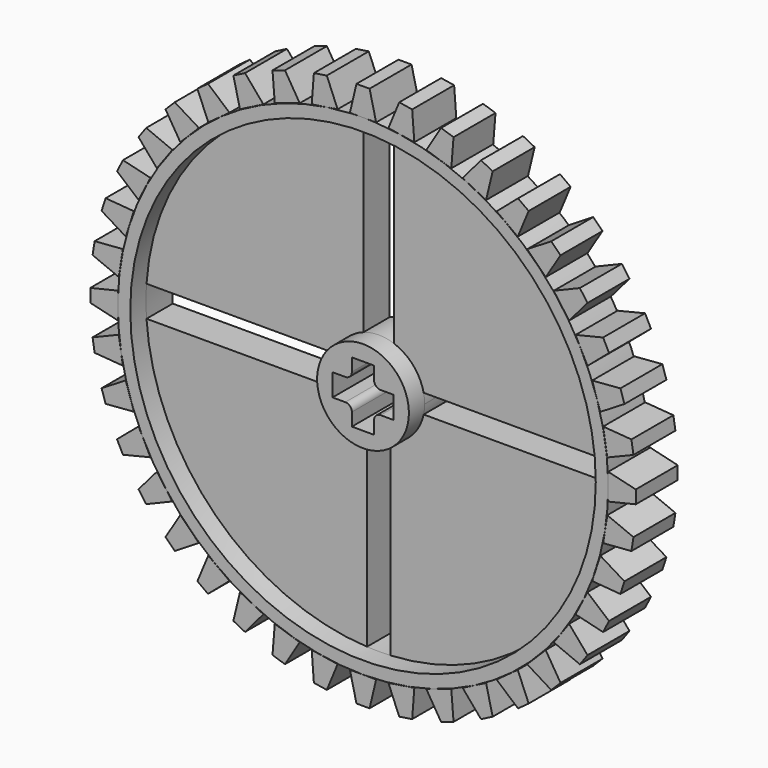
from build123d import *

# Parameters (mm, degrees)
F1_DEPTH        = 4
F2_DEPTH        = 4
F2_COPIES_COUNT = 40
F3_W            = 1.475
F3_H            = 1.693
F3_W_2          = 1.693
F3_H_2          = 1.4767124441
F3_W_3          = 1.482
F3_H_3          = 1.4802875559
F4_DEPTH        = 25
F5_R            = 17.75
F5_R_2          = 3.5
F6_DEPTH        = 0.75
F7_R            = 17.75
F7_R_2          = 3.5
F8_DEPTH        = 0.75
F9_R            = 0.5
F11_DEPTH       = 25


# Not quite as in the source:
# - after a boolean that leaves OpenCascade's solid faulty, fix() repairs it
# - a pattern or mirror of a feature is missing from the dataset's text; its kind, count and spacing are read off the source's solid


with BuildPart() as f1:
    # F0 (on Front) → F1 (new body)
    with BuildSketch(Plane.XZ):
        with BuildLine():
            ThreePointArc((-1.0015409707, 18.6731603025), (-12.8639259919, -13.5723766554), (18.7, 0))
            ThreePointArc((18.7, 0), (13.571937199, 12.8643896344), (1.0002651695, 18.6732286868))
            ThreePointArc((1.0002651695, 18.6732286868), (0.500311681, 18.6933059736), (0, 18.7))
            ThreePointArc((0, 18.7), (-0.5009502683, 18.6932888714), (-1.0015409707, 18.6731603025))
        make_face()
    extrude(amount=F1_DEPTH)

    # F3 (on face) → F4 (cut)
    with BuildSketch(Plane.XZ.offset(4)):
        with Locations((-1.5875, 0.0017875559)):
            Rectangle(F3_W, F3_H)
        with Locations((-0.0035, 1.5866437779)):
            Rectangle(F3_W_2, F3_H_2)
        with Locations((-0.0035, 0.0017875559)):
            Rectangle(F3_W_2, F3_H)
        with Locations((1.584, 0.0017875559)):
            Rectangle(F3_W_3, F3_H)
        with Locations((-0.0035, -1.5848562221)):
            Rectangle(F3_W_2, F3_H_3)
    extrude(amount=-F4_DEPTH, mode=Mode.SUBTRACT)

    # F5 (on face) → F6 (cut)
    with BuildSketch(Plane.XZ.offset(4)):
        Circle(F5_R)
        Circle(F5_R_2, mode=Mode.SUBTRACT)
    extrude(amount=-F6_DEPTH, mode=Mode.SUBTRACT)

    # F7 (on face) → F8 (cut)
    with BuildSketch(Plane.XZ.offset(3.25)):
        Circle(F7_R)
        Circle(F7_R_2, mode=Mode.SUBTRACT)
    extrude(amount=-F8_DEPTH, mode=Mode.SUBTRACT)

    # F9
    f9_edges = [f1.edges().sort_by_distance(p)[0] for p in [
        (-0.85, -2, 0.848288),
        (0.843, -2, 0.848288),
        (-0.85, -2, -0.844712),
        (0.843, -2, -0.844712),
    ]]
    fillet(f9_edges, radius=F9_R)

    # F10 (on face) → F11 (cut)
    with BuildSketch(Plane.XZ.offset(2.5)):
        with BuildLine():
            ThreePointArc((-3.2968505322, -1.1750644953), (-3.5, 0), (-3.2968505322, 1.1750644953))
            Line((-3.2968505322, 1.1750644953), (-17.7110621768, 1.1750644953))
            ThreePointArc((-17.7110621768, 1.1750644953), (-17.75, 0), (-17.7110621768, -1.1750644953))
            Line((-17.7110621768, -1.1750644953), (-3.2968505322, -1.1750644953))
        make_face()
        with BuildLine():
            Line((0.8961235281, -17.7273647963), (0.8961235281, -3.3833360197))
            ThreePointArc((0.8961235281, -3.3833360197), (0, -3.5), (-0.8961235281, -3.3833360197))
            Line((-0.8961235281, -3.3833360197), (-0.8961235281, -17.7273647963))
            ThreePointArc((-0.8961235281, -17.7273647963), (0, -17.75), (0.8961235281, -17.7273647963))
        make_face()
        with BuildLine():
            Line((17.7349775585, 0.7301171139), (3.423, 0.7301171139))
            ThreePointArc((3.423, 0.7301171139), (3.4806967693, 0.3670830969), (3.5, 0))
            ThreePointArc((3.5, 0), (3.4806967693, -0.3670830969), (3.423, -0.7301171139))
            Line((3.423, -0.7301171139), (17.7349775585, -0.7301171139))
            ThreePointArc((17.7349775585, -0.7301171139), (17.7462439922, -0.3651358219), (17.75, 0))
            ThreePointArc((17.75, 0), (17.7462439922, 0.3651358219), (17.7349775585, 0.7301171139))
        make_face()
        with BuildLine():
            ThreePointArc((-1.163931855, 3.3007972729), (0, 3.5), (1.163931855, 3.3007972729))
            Line((1.163931855, 3.3007972729), (1.163931855, 17.7117972729))
            ThreePointArc((1.163931855, 17.7117972729), (0, 17.75), (-1.163931855, 17.7117972729))
            Line((-1.163931855, 17.7117972729), (-1.163931855, 3.3007972729))
        make_face()
    extrude(amount=-F11_DEPTH, mode=Mode.SUBTRACT)

    add(f1.part.fix(), mode=Mode.REPLACE)


with BuildPart() as f2:
    # F0 (on Front) → F2 (new body)
    with BuildSketch(Plane.XZ):
        Polygon((-1, 18.7), (0, 18.7), (0, 20.8), (-0.5, 20.8), align=None)
        Polygon((0, 20.8), (0, 18.7), (1, 18.7), (0.5, 20.8), align=None)
    extrude(amount=F2_DEPTH)


with BuildPart() as f2_copies_1:
    # F2_copies: instance of F2
    add(f2.part.rotate(Axis((0, 0, 0), (0, 1, 0)), 1 * 360 / F2_COPIES_COUNT))


with BuildPart() as f2_copies_2:
    # F2_copies: instance of F2
    add(f2.part.rotate(Axis((0, 0, 0), (0, 1, 0)), 2 * 360 / F2_COPIES_COUNT))


with BuildPart() as f2_copies_3:
    # F2_copies: instance of F2
    add(f2.part.rotate(Axis((0, 0, 0), (0, 1, 0)), 3 * 360 / F2_COPIES_COUNT))


with BuildPart() as f2_copies_4:
    # F2_copies: instance of F2
    add(f2.part.rotate(Axis((0, 0, 0), (0, 1, 0)), 4 * 360 / F2_COPIES_COUNT))


with BuildPart() as f2_copies_5:
    # F2_copies: instance of F2
    add(f2.part.rotate(Axis((0, 0, 0), (0, 1, 0)), 5 * 360 / F2_COPIES_COUNT))


with BuildPart() as f2_copies_6:
    # F2_copies: instance of F2
    add(f2.part.rotate(Axis((0, 0, 0), (0, 1, 0)), 6 * 360 / F2_COPIES_COUNT))


with BuildPart() as f2_copies_7:
    # F2_copies: instance of F2
    add(f2.part.rotate(Axis((0, 0, 0), (0, 1, 0)), 7 * 360 / F2_COPIES_COUNT))


with BuildPart() as f2_copies_8:
    # F2_copies: instance of F2
    add(f2.part.rotate(Axis((0, 0, 0), (0, 1, 0)), 8 * 360 / F2_COPIES_COUNT))


with BuildPart() as f2_copies_9:
    # F2_copies: instance of F2
    add(f2.part.rotate(Axis((0, 0, 0), (0, 1, 0)), 9 * 360 / F2_COPIES_COUNT))


with BuildPart() as f2_copies_10:
    # F2_copies: instance of F2
    add(f2.part.rotate(Axis((0, 0, 0), (0, 1, 0)), 10 * 360 / F2_COPIES_COUNT))


with BuildPart() as f2_copies_11:
    # F2_copies: instance of F2
    add(f2.part.rotate(Axis((0, 0, 0), (0, 1, 0)), 11 * 360 / F2_COPIES_COUNT))


with BuildPart() as f2_copies_12:
    # F2_copies: instance of F2
    add(f2.part.rotate(Axis((0, 0, 0), (0, 1, 0)), 12 * 360 / F2_COPIES_COUNT))


with BuildPart() as f2_copies_13:
    # F2_copies: instance of F2
    add(f2.part.rotate(Axis((0, 0, 0), (0, 1, 0)), 13 * 360 / F2_COPIES_COUNT))


with BuildPart() as f2_copies_14:
    # F2_copies: instance of F2
    add(f2.part.rotate(Axis((0, 0, 0), (0, 1, 0)), 14 * 360 / F2_COPIES_COUNT))


with BuildPart() as f2_copies_15:
    # F2_copies: instance of F2
    add(f2.part.rotate(Axis((0, 0, 0), (0, 1, 0)), 15 * 360 / F2_COPIES_COUNT))


with BuildPart() as f2_copies_16:
    # F2_copies: instance of F2
    add(f2.part.rotate(Axis((0, 0, 0), (0, 1, 0)), 16 * 360 / F2_COPIES_COUNT))


with BuildPart() as f2_copies_17:
    # F2_copies: instance of F2
    add(f2.part.rotate(Axis((0, 0, 0), (0, 1, 0)), 17 * 360 / F2_COPIES_COUNT))


with BuildPart() as f2_copies_18:
    # F2_copies: instance of F2
    add(f2.part.rotate(Axis((0, 0, 0), (0, 1, 0)), 18 * 360 / F2_COPIES_COUNT))


with BuildPart() as f2_copies_19:
    # F2_copies: instance of F2
    add(f2.part.rotate(Axis((0, 0, 0), (0, 1, 0)), 19 * 360 / F2_COPIES_COUNT))


with BuildPart() as f2_copies_20:
    # F2_copies: instance of F2
    add(f2.part.rotate(Axis((0, 0, 0), (0, 1, 0)), 20 * 360 / F2_COPIES_COUNT))


with BuildPart() as f2_copies_21:
    # F2_copies: instance of F2
    add(f2.part.rotate(Axis((0, 0, 0), (0, 1, 0)), 21 * 360 / F2_COPIES_COUNT))


with BuildPart() as f2_copies_22:
    # F2_copies: instance of F2
    add(f2.part.rotate(Axis((0, 0, 0), (0, 1, 0)), 22 * 360 / F2_COPIES_COUNT))


with BuildPart() as f2_copies_23:
    # F2_copies: instance of F2
    add(f2.part.rotate(Axis((0, 0, 0), (0, 1, 0)), 23 * 360 / F2_COPIES_COUNT))


with BuildPart() as f2_copies_24:
    # F2_copies: instance of F2
    add(f2.part.rotate(Axis((0, 0, 0), (0, 1, 0)), 24 * 360 / F2_COPIES_COUNT))


with BuildPart() as f2_copies_25:
    # F2_copies: instance of F2
    add(f2.part.rotate(Axis((0, 0, 0), (0, 1, 0)), 25 * 360 / F2_COPIES_COUNT))


with BuildPart() as f2_copies_26:
    # F2_copies: instance of F2
    add(f2.part.rotate(Axis((0, 0, 0), (0, 1, 0)), 26 * 360 / F2_COPIES_COUNT))


with BuildPart() as f2_copies_27:
    # F2_copies: instance of F2
    add(f2.part.rotate(Axis((0, 0, 0), (0, 1, 0)), 27 * 360 / F2_COPIES_COUNT))


with BuildPart() as f2_copies_28:
    # F2_copies: instance of F2
    add(f2.part.rotate(Axis((0, 0, 0), (0, 1, 0)), 28 * 360 / F2_COPIES_COUNT))


with BuildPart() as f2_copies_29:
    # F2_copies: instance of F2
    add(f2.part.rotate(Axis((0, 0, 0), (0, 1, 0)), 29 * 360 / F2_COPIES_COUNT))


with BuildPart() as f2_copies_30:
    # F2_copies: instance of F2
    add(f2.part.rotate(Axis((0, 0, 0), (0, 1, 0)), 30 * 360 / F2_COPIES_COUNT))


with BuildPart() as f2_copies_31:
    # F2_copies: instance of F2
    add(f2.part.rotate(Axis((0, 0, 0), (0, 1, 0)), 31 * 360 / F2_COPIES_COUNT))


with BuildPart() as f2_copies_32:
    # F2_copies: instance of F2
    add(f2.part.rotate(Axis((0, 0, 0), (0, 1, 0)), 32 * 360 / F2_COPIES_COUNT))


with BuildPart() as f2_copies_33:
    # F2_copies: instance of F2
    add(f2.part.rotate(Axis((0, 0, 0), (0, 1, 0)), 33 * 360 / F2_COPIES_COUNT))


with BuildPart() as f2_copies_34:
    # F2_copies: instance of F2
    add(f2.part.rotate(Axis((0, 0, 0), (0, 1, 0)), 34 * 360 / F2_COPIES_COUNT))


with BuildPart() as f2_copies_35:
    # F2_copies: instance of F2
    add(f2.part.rotate(Axis((0, 0, 0), (0, 1, 0)), 35 * 360 / F2_COPIES_COUNT))


with BuildPart() as f2_copies_36:
    # F2_copies: instance of F2
    add(f2.part.rotate(Axis((0, 0, 0), (0, 1, 0)), 36 * 360 / F2_COPIES_COUNT))


with BuildPart() as f2_copies_37:
    # F2_copies: instance of F2
    add(f2.part.rotate(Axis((0, 0, 0), (0, 1, 0)), 37 * 360 / F2_COPIES_COUNT))


with BuildPart() as f2_copies_38:
    # F2_copies: instance of F2
    add(f2.part.rotate(Axis((0, 0, 0), (0, 1, 0)), 38 * 360 / F2_COPIES_COUNT))


with BuildPart() as f2_copies_39:
    # F2_copies: instance of F2
    add(f2.part.rotate(Axis((0, 0, 0), (0, 1, 0)), 39 * 360 / F2_COPIES_COUNT))


solid = Compound([f1.part, f2.part, f2_copies_1.part, f2_copies_2.part, f2_copies_3.part, f2_copies_4.part, f2_copies_5.part, f2_copies_6.part, f2_copies_7.part, f2_copies_8.part, f2_copies_9.part, f2_copies_10.part, f2_copies_11.part, f2_copies_12.part, f2_copies_13.part, f2_copies_14.part, f2_copies_15.part, f2_copies_16.part, f2_copies_17.part, f2_copies_18.part, f2_copies_19.part, f2_copies_20.part, f2_copies_21.part, f2_copies_22.part, f2_copies_23.part, f2_copies_24.part, f2_copies_25.part, f2_copies_26.part, f2_copies_27.part, f2_copies_28.part, f2_copies_29.part, f2_copies_30.part, f2_copies_31.part, f2_copies_32.part, f2_copies_33.part, f2_copies_34.part, f2_copies_35.part, f2_copies_36.part, f2_copies_37.part, f2_copies_38.part, f2_copies_39.part])
